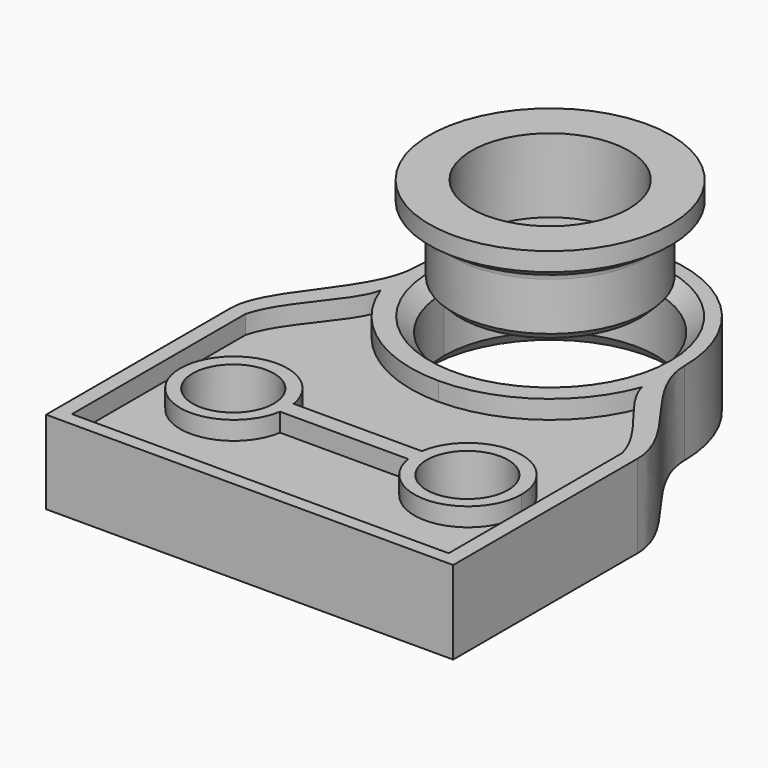
from build123d import *

# Parameters (mm, degrees)
F0_R      = 4.25
F0_R_2    = 3.05
F1_DEPTH  = 1
F0_R_3    = 5.25
F2_DEPTH  = 5
F3_SIZE   = 0.4
F5_R      = 6.5245521105
F5_R_2    = 4.8436348364
F6_DEPTH  = 1.5
F7_R      = 0.5
F8_SIZE2  = 0.7140740034
F8_SIZE   = 0.5
F10_R     = 2.2
F11_DEPTH = 4.5
F15_DEPTH = 1


# Not quite as in the source:
# - a fillet or chamfer that OpenCascade refuses, or shapes differently, is made with other operations: its cross-section is extruded or revolved along the edge and cut away or added


with BuildPart() as f1:
    # F0 (on Top) → F1 (new body)
    with BuildSketch(Plane.XY):
        Circle(F0_R)
        Circle(F0_R_2, mode=Mode.SUBTRACT)
    extrude(amount=F1_DEPTH)

    # F0 (on Top) → F2 (join)
    with BuildSketch(Plane.XY):
        Circle(F0_R_3)
        Circle(F0_R, mode=Mode.SUBTRACT)
    extrude(amount=F2_DEPTH)

    # F3
    f3_edges = [f1.edges().sort_by_distance(p)[0] for p in [
        (-5.25, 0, 0),
    ]]
    chamfer(f3_edges, length=F3_SIZE)

    # F5 (on offset) → F6 (join)
    with BuildSketch(Plane.XY.offset(5)):
        Circle(F5_R)
        Circle(F5_R_2, mode=Mode.SUBTRACT)
    extrude(amount=-F6_DEPTH)

    # F7
    f7_edges = [f1.edges().sort_by_distance(p)[0] for p in [
        (-5.25, 0, 3.5),
    ]]
    fillet(f7_edges, radius=F7_R)

    # F8
    f8_edges = [f1.edges().sort_by_distance(p)[0] for p in [
        (-6.524552, 0, 3.5),
    ]]
    f8_side = f1.faces().sort_by_distance((-6.524552, 0, 4.25))[0]
    chamfer(f8_edges, length=F8_SIZE, length2=F8_SIZE2, reference=f8_side)


with BuildPart() as f11:
    # F10 (on offset) → F11 (new body)
    with BuildSketch(Plane.XY.offset(-6)):
        with BuildLine():
            ThreePointArc((-5.75, 0), (0, 5.75), (5.75, 0))
            Line((5.75, 0), (7.25, 0))
            ThreePointArc((7.25, 0), (0, 7.25), (-7.25, 0))
            Line((-7.25, 0), (-5.75, 0))
        make_face()
        with BuildLine():
            ThreePointArc((-4.3594842183, -3.749319585), (-5.3911749302, -1.9994331378), (-5.75, 0))
            Line((-5.75, 0), (-7.25, 0))
            ThreePointArc((-7.25, 0), (-6.9839296942, -1.9460796559), (-6.2052479926, -3.749319585))
            Line((-6.2052479926, -3.749319585), (-4.3594842183, -3.749319585))
        make_face()
        with BuildLine():
            Line((6.2052479926, -3.749319585), (4.3594842183, -3.749319585))
            ThreePointArc((4.3594842183, -3.749319585), (0, -5.75), (-4.3594842183, -3.749319585))
            Line((-4.3594842183, -3.749319585), (-6.2052479926, -3.749319585))
            ThreePointArc((-6.2052479926, -3.749319585), (0, -7.25), (6.2052479926, -3.749319585))
        make_face()
        with BuildLine():
            Line((7.25, 0), (5.75, 0))
            ThreePointArc((5.75, 0), (5.3911749302, -1.9994331378), (4.3594842183, -3.749319585))
            Line((4.3594842183, -3.749319585), (6.2052479926, -3.749319585))
            ThreePointArc((6.2052479926, -3.749319585), (6.9839296942, -1.9460796559), (7.25, 0))
        make_face()
        with BuildLine():
            ThreePointArc((-6.2052479926, -3.749319585), (-6.9839296942, -1.9460796559), (-7.25, 0))
            add(Edge.make_bspline(
                [(-7.25, 0), (-7.2656506928, -1.3271520952), (-8.0546621033, -2.5618388367), (-8.9048569039, -3.749319585)],
                knots=[0, 0, 0, 0, 3.981709245, 3.981709245, 3.981709245, 3.981709245], degree=3))
            Line((-8.9048569039, -3.749319585), (-6.2052479926, -3.749319585))
        make_face()
        with BuildLine():
            Line((8.9863599272, -3.749319585), (6.2052479926, -3.749319585))
            ThreePointArc((6.2052479926, -3.749319585), (0, -7.25), (-6.2052479926, -3.749319585))
            Line((-6.2052479926, -3.749319585), (-8.9048569039, -3.749319585))
            add(Edge.make_bspline(
                [(-8.9048569039, -3.749319585), (-9.9096958288, -5.1527942681), (-11, -6.4903283123), (-11, -7.8366426751)],
                knots=[3.981709245, 3.981709245, 3.981709245, 3.981709245, 8.6876618498, 8.6876618498, 8.6876618498, 8.6876618498], degree=3))
            Line((-11, -7.8366426751), (11, -7.8366426751))
            add(Edge.make_bspline(
                [(8.9863599272, -3.749319585), (9.9677269971, -5.1019814592), (11, -6.4384359832), (11, -7.8366426751)],
                knots=[4.1157167981, 4.1157167981, 4.1157167981, 4.1157167981, 8.6876618498, 8.6876618498, 8.6876618498, 8.6876618498], degree=3))
        make_face()
        with BuildLine():
            add(Edge.make_bspline(
                [(7.25, 0), (7.2607375636, -1.3008223386), (8.1029221586, -2.5316380218), (8.9863599272, -3.749319585)],
                knots=[0, 0, 0, 0, 4.1157167981, 4.1157167981, 4.1157167981, 4.1157167981], degree=3))
            ThreePointArc((7.25, 0), (6.9839296942, -1.9460796559), (6.2052479926, -3.749319585))
            Line((6.2052479926, -3.749319585), (8.9863599272, -3.749319585))
        make_face()
        Polygon((11, -20.3), (11, -7.8366426751), (-11, -7.8366426751), (-11, -20.3), (0, -20.3), align=None)
        with Locations((-6.325, -13.4990205988)):
            Circle(F10_R, mode=Mode.SUBTRACT)
        with BuildLine():
            ThreePointArc((8.525, -13.4990205988), (6.325, -15.6990205988), (4.125, -13.4990205988))
            ThreePointArc((4.125, -13.4990205988), (6.325, -11.2990205988), (8.525, -13.4990205988))
        make_face(mode=Mode.SUBTRACT)
    extrude(amount=F11_DEPTH)

    # F12: chamfer of 0.75 on 2 edges, made by hand

    # F12_s1 → F12_t2 (revolve, cut)
    with BuildSketch(Plane.XZ):
        Polygon((5.75, -2.25), (6.5, -1.5), (5.75, -1.5), align=None)
    revolve(axis=Axis((0, 0, -1.5), (0, 0, -1)), mode=Mode.SUBTRACT)

    # F12_s3 → F12_t4 (revolve, cut)
    with BuildSketch(Plane.XZ):
        Polygon((5.75, -5.25), (6.5, -6), (5.75, -6), align=None)
    revolve(axis=Axis((0, 0, -6), (0, 0, -1)), mode=Mode.SUBTRACT)

    # F14 (on offset) → F15 (cut)
    with BuildSketch(Plane.XY.offset(-1.5)):
        with BuildLine():
            ThreePointArc((0, -7.5402029312), (-4.3061145714, -6.1896718444), (-7.0696866821, -2.6218677427))
            add(Edge.make_bspline(
                [(-10.1782370821, -7.8539925324), (-9.6560776489, -5.8711635466), (-7.4144124978, -4.1833631916), (-7.0696866821, -2.6218677427)],
                knots=[0, 0, 0, 0, 6.0859030065, 6.0859030065, 6.0859030065, 6.0859030065], degree=3))
            Line((-10.1782370821, -7.8539925324), (-10.1782370821, -19.5775783759))
            Line((-10.1782370821, -19.5775783759), (0, -19.5775783759))
            Line((0, -19.5775783759), (0, -13.9200452533))
            Line((0, -13.9200452533), (-3.4618476619, -13.9200452533))
            ThreePointArc((-3.4618476619, -13.9200452533), (-9.2249834149, -13.4591182958), (-3.4618476619, -12.9981913384))
            Line((-3.4618476619, -12.9981913384), (0, -12.9981913384))
            Line((0, -12.9981913384), (0, -7.5402029312))
        make_face()
        with BuildLine():
            add(Edge.make_bspline(
                [(10.1782370821, -7.8539925324), (9.6560776489, -5.8711635466), (7.4144124978, -4.1833631916), (7.0696866821, -2.6218677427)],
                knots=[0, 0, 0, 0, 6.0859030065, 6.0859030065, 6.0859030065, 6.0859030065], degree=3))
            ThreePointArc((7.0696866821, -2.6218677427), (4.3061145714, -6.1896718444), (0, -7.5402029312))
            Line((0, -7.5402029312), (0, -12.9981913384))
            Line((0, -12.9981913384), (3.461807566, -12.9981913384))
            ThreePointArc((3.461807566, -12.9981913384), (6.5559861293, -10.5678753889), (9.225016577, -13.4586630092))
            ThreePointArc((9.225016577, -13.4586630092), (6.5564458102, -16.3494138649), (3.4619541562, -13.9200452533))
            Line((3.4619541562, -13.9200452533), (0, -13.9200452533))
            Line((0, -13.9200452533), (0, -19.5775783759))
            Line((0, -19.5775783759), (10.1782370821, -19.5775783759))
            Line((10.1782370821, -19.5775783759), (10.1782370821, -7.8539925324))
        make_face()
    extrude(amount=-F15_DEPTH, mode=Mode.SUBTRACT)


solid = Compound([f1.part, f11.part])
